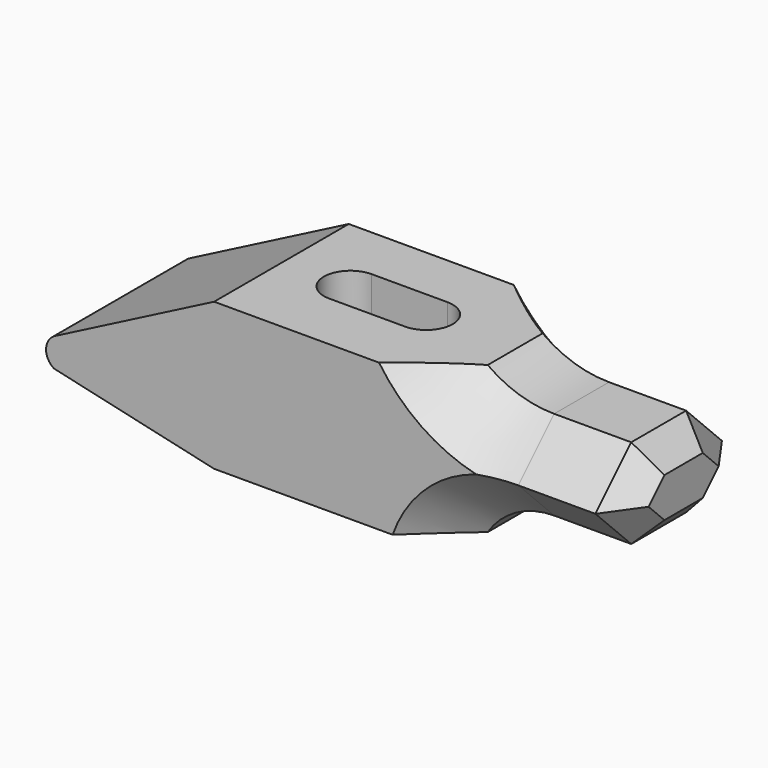
from build123d import *

# Parameters (mm, degrees)
F1_DEPTH     = 34.29
F2_T1_DEPTH  = 46.9101181819
F2_T4_ANGLE  = 100.0995199097
F2_T6_ANGLE  = 150.1003280787
F2_T8_ANGLE  = 150.1003280787
F2_T10_ANGLE = 100.0995199097
F4_DEPTH     = 64.008
F5_SIZE      = 5.08


# Not quite as in the source:
# - a fillet or chamfer that OpenCascade refuses, or shapes differently, is made with other operations: its cross-section is extruded or revolved along the edge and cut away or added


with BuildPart() as f1:
    # F0 (on Front) → F1 (new body)
    with BuildSketch(Plane.XZ):
        with BuildLine():
            Line((23.1983069149, 22.5941853283), (-24.4065547209, 22.5941853283))
            Line((-24.4065547209, 22.5941853283), (-56.7875248861, 5.9204018954))
            ThreePointArc((-56.7875248861, 5.9204018954), (-58.6318372817, 3.0305487818), (-57.02917908, 0))
            Line((-57.02917908, 0), (-24.4065547209, -7.3702961741))
            Line((-24.4065547209, -7.3702961741), (23.1983069149, -7.3702961741))
            ThreePointArc((23.1983069149, -7.3702961741), (29.0260188517, -1.9620688543), (36.7306560898, 0))
            Line((36.7306560898, 0), (57.5124751139, 0))
            Line((57.5124751139, 0), (57.5124751139, 18.2445040364))
            Line((57.5124751139, 18.2445040364), (36.7306560898, 18.2445040364))
            ThreePointArc((36.7306560898, 18.2445040364), (29.6235434283, 19.3586478737), (23.1983069149, 22.5941853283))
        make_face()
    extrude(amount=F1_DEPTH)

    # F2: chamfer of 10.16 on 4 edges, made by hand

    # F2_s2 → F2_t1 (cut)
    with BuildSketch(Plane.YZ.offset(36.7306560898)):
        Polygon((-24.13, 18.2445040364), (-34.29, 8.0845040364), (-34.29, 18.2445040364), align=None)
        Polygon((-24.13, 0), (-34.29, 10.16), (-34.29, 0), align=None)
        Polygon((-10.16, 0), (0, 10.16), (0, 0), align=None)
        Polygon((-10.16, 18.2445040364), (0, 8.0845040364), (0, 18.2445040364), align=None)
    extrude(amount=F2_T1_DEPTH, mode=Mode.SUBTRACT)

    # F2_s3 → F2_t4 (revolve, cut)
    with BuildSketch(Plane.YZ.offset(36.7306560898)):
        Polygon((-10.16, 18.2445040364), (0, 8.0845040364), (0, 18.2445040364), align=None)
    revolve(axis=Axis((36.7306560898, 0, 41.469677098), (0, 1, 0)), revolution_arc=F2_T4_ANGLE, mode=Mode.SUBTRACT)

    # F2_s5 → F2_t6 (revolve, cut)
    with BuildSketch(Plane(origin=(34.5645844349, 0, -19.8752542161), x_dir=(0, 1, 0), z_dir=(0.8668996033, 0, -0.4984827758))):
        Polygon((-10.16, -11.7629612563), (0, -21.9229612563), (0, -11.7629612563), align=None)
    revolve(axis=Axis((36.7306560898, 0, -16.1082902421), (0, 1, 0)), revolution_arc=F2_T6_ANGLE, mode=Mode.SUBTRACT)

    # F2_s7 → F2_t8 (revolve, cut)
    with BuildSketch(Plane(origin=(34.5645844349, 0, -19.8752542161), x_dir=(0, 1, 0), z_dir=(0.8668996033, 0, -0.4984827758))):
        Polygon((-24.13, -11.7629612563), (-34.29, -21.9229612563), (-34.29, -11.7629612563), align=None)
    revolve(axis=Axis((36.7306560898, -34.29, -16.1082902421), (0, 1, 0)), revolution_arc=F2_T8_ANGLE, mode=Mode.SUBTRACT)

    # F2_s9 → F2_t10 (revolve, cut)
    with BuildSketch(Plane.YZ.offset(36.7306560898)):
        Polygon((-24.13, 18.2445040364), (-34.29, 8.0845040364), (-34.29, 18.2445040364), align=None)
    revolve(axis=Axis((36.7306560898, -34.29, 41.469677098), (0, 1, 0)), revolution_arc=F2_T10_ANGLE, mode=Mode.SUBTRACT)

    # F3 (on Top) → F4 (cut)
    with BuildSketch(Plane.XY):
        with BuildLine():
            Line((4.6636075713, -11.2218027934), (-10.7845906168, -11.2218027934))
            ThreePointArc((-10.7845906168, -11.2218027934), (-16.1768863909, -16.6140985675), (-10.7845906168, -22.0063943416))
            Line((-10.7845906168, -22.0063943416), (4.6636075713, -22.0063943416))
            ThreePointArc((4.6636075713, -22.0063943416), (10.0559033453, -16.6140985675), (4.6636075713, -11.2218027934))
        make_face()
    extrude(amount=F4_DEPTH, mode=Mode.SUBTRACT)

    # F5
    f5_edges = [f1.edges().sort_by_distance(p)[0] for p in [
        (57.512475, -28.691126, 13.683378),
        (57.512475, -17.145, 18.244504),
        (57.512475, -5.598874, 13.683378),
        (57.512475, -17.145, 0),
        (57.512475, -28.691126, 4.561126),
        (57.512475, -5.598874, 4.561126),
    ]]
    chamfer(f5_edges, length=F5_SIZE)


solid = f1.part
